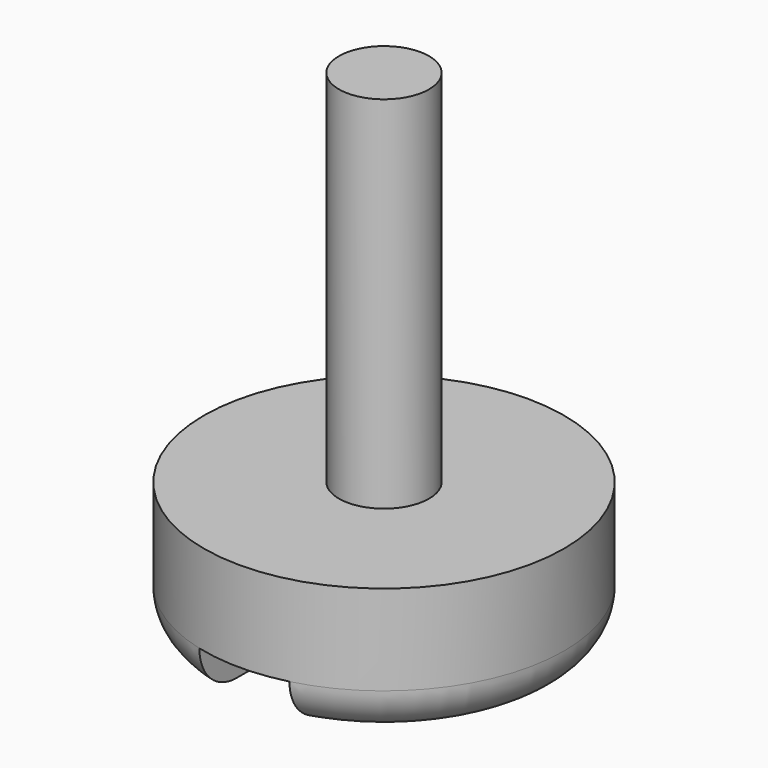
from build123d import *

# Parameters (mm, degrees)
F0_R     = 4
F1_DEPTH = 3
F2_R     = 1
F3_DEPTH = 8
F4_W     = 2
F4_H     = 10.9652710235
F5_DEPTH = 1
F6_R     = 1


with BuildPart() as f1:
    # F0 (on Top) → F1 (new body)
    with BuildSketch(Plane.XY):
        Circle(F0_R)
    extrude(amount=F1_DEPTH)

    # F2 (on face) → F3 (join)
    with BuildSketch(Plane.XY.offset(3)):
        Circle(F2_R)
    extrude(amount=F3_DEPTH)

    # F4 (on face) → F5 (cut)
    with BuildSketch(Plane(origin=(0, 0, 0), x_dir=(1, 0, 0), z_dir=(0, 0, -1))):
        Rectangle(F4_W, F4_H)
    extrude(amount=-F5_DEPTH, mode=Mode.SUBTRACT)

    # F6
    f6_edges = [f1.edges().sort_by_distance(p)[0] for p in [
        (-4, 0, 0),
        (3.162278, 2.44949, 0),
        (3.162278, -2.44949, 0),
    ]]
    fillet(f6_edges, radius=F6_R)


solid = f1.part
